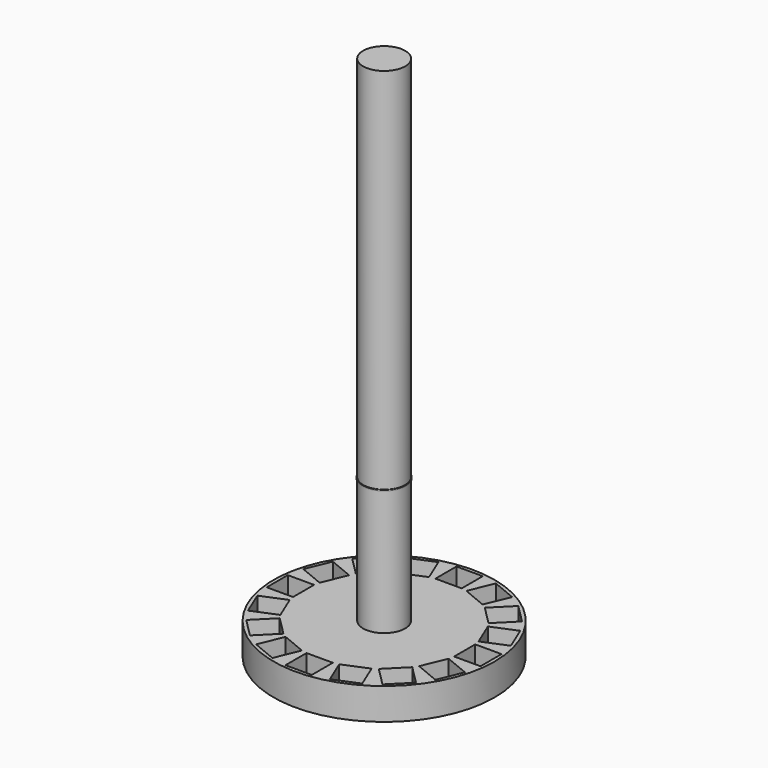
from build123d import *

# Parameters (mm, degrees)
F0_W     = 21
F0_H     = 6
F2_R     = 4
F3_DEPTH = 100
F4_W     = 5
F4_H     = 5
F5_DEPTH = 5.4
F6_W     = 4.1
F6_H     = 0.2


# Not quite as in the source:
# - a feature names something its author has since deleted; it is built from what else it names


with BuildPart() as f1:
    # F0 (on Front) → F1 (revolve)
    with BuildSketch(Plane.XZ):
        with Locations((10.5, 3)):
            Rectangle(F0_W, F0_H)
    revolve(axis=Axis((0, 0, 3), (0, 0, -1)))

    # F2 (on Top) → F3 (join)
    with BuildSketch(Plane.XY):
        Circle(F2_R)
    extrude(amount=F3_DEPTH)

    # F4 (on face) → F5 (cut)
    with BuildSketch(Plane.XY.offset(6)):
        with Locations((0, 17.8)):
            Rectangle(F4_W, F4_H)
        Polygon((-8.1647553465, 13.1786482665), (-3.5453576839, 15.0920654283), (-5.4587748457, 19.7114630909), (-10.0781725083, 17.7980459291), align=None)
        Polygon((3.5453576839, 15.0920654283), (8.1647553465, 13.1786482665), (10.0781725083, 17.7980459291), (5.4587748457, 19.7114630909), align=None)
        Polygon((9.0509667992, 12.5865007051), (12.5865007051, 9.0509667992), (16.1220346111, 12.5865007051), (12.5865007051, 16.1220346111), align=None)
        Polygon((13.1786482665, 8.1647553465), (15.0920654283, 3.5453576839), (19.7114630909, 5.4587748457), (17.7980459291, 10.0781725083), align=None)
        with Locations((17.8, 0)):
            Rectangle(F4_W, F4_H)
        Polygon((15.0920654283, -3.5453576839), (13.1786482665, -8.1647553465), (17.7980459291, -10.0781725083), (19.7114630909, -5.4587748457), align=None)
        Polygon((12.5865007051, -9.0509667992), (9.0509667992, -12.5865007051), (12.5865007051, -16.1220346111), (16.1220346111, -12.5865007051), align=None)
        Polygon((-12.5865007051, 9.0509667992), (-9.0509667992, 12.5865007051), (-12.5865007051, 16.1220346111), (-16.1220346111, 12.5865007051), align=None)
        Polygon((-15.0920654283, 3.5453576839), (-13.1786482665, 8.1647553465), (-17.7980459291, 10.0781725083), (-19.7114630909, 5.4587748457), align=None)
        with Locations((-17.8, 0)):
            Rectangle(F4_W, F4_H)
        Polygon((-13.1786482665, -8.1647553465), (-15.0920654283, -3.5453576839), (-19.7114630909, -5.4587748457), (-17.7980459291, -10.0781725083), align=None)
        Polygon((-9.0509667992, -12.5865007051), (-12.5865007051, -9.0509667992), (-16.1220346111, -12.5865007051), (-12.5865007051, -16.1220346111), align=None)
        Polygon((-3.5453576839, -15.0920654283), (-8.1647553465, -13.1786482665), (-10.0781725083, -17.7980459291), (-5.4587748457, -19.7114630909), align=None)
        with Locations((0, -17.8)):
            Rectangle(F4_W, F4_H)
        Polygon((8.1647553465, -13.1786482665), (3.5453576839, -15.0920654283), (5.4587748457, -19.7114630909), (10.0781725083, -17.7980459291), align=None)
    extrude(amount=-F5_DEPTH, mode=Mode.SUBTRACT)

    # F6 (on Right) → F7 (revolve)
    with BuildSketch(Plane.YZ):
        with Locations((2.05, 29.9)):
            Rectangle(F6_W, F6_H)
    revolve(axis=Axis((0, 0, 29.9), (0, 0, -1)))


solid = f1.part
